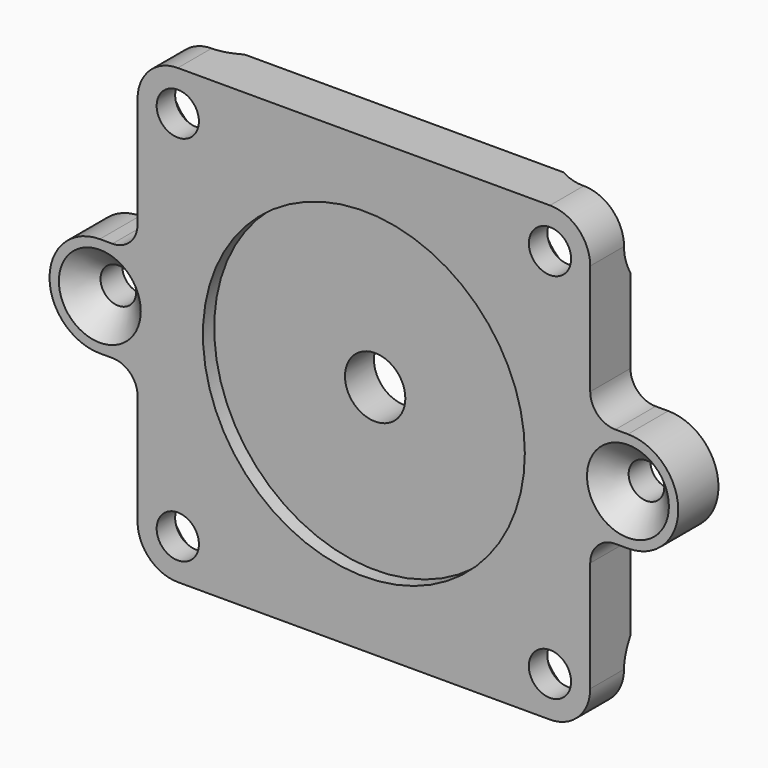
from build123d import *

# Parameters (mm, degrees)
F0_R     = 2.667
F0_R_2   = 2.2479
F0_R_3   = 3.81
F1_DEPTH = 6.35
F2_R     = 20.32
F2_R_2   = 3.81
F3_DEPTH = 1.778
F4_SIZE  = 2.921


# Not quite as in the source:
# - a fillet or chamfer that OpenCascade refuses, or shapes differently, is made with other operations: its cross-section is extruded or revolved along the edge and cut away or added


with BuildPart() as f1:
    # F0 (on Front) → F1 (new body)
    with BuildSketch(Plane.XZ):
        with BuildLine():
            Line((-23.495, -28.575), (23.495, -28.575))
            ThreePointArc((23.495, -28.575), (27.0871024484, -27.0871024484), (28.575, -23.495))
            Line((28.575, -23.495), (28.575, -9.525))
            ThreePointArc((28.575, -9.525), (29.5049359697, -7.2799359697), (31.75, -6.35))
            Line((31.75, -6.35), (33.3375, -6.35))
            ThreePointArc((33.3375, -6.35), (39.6875, 0), (33.3375, 6.35))
            Line((33.3375, 6.35), (31.75, 6.35))
            ThreePointArc((31.75, 6.35), (29.5049359697, 7.2799359697), (28.575, 9.525))
            Line((28.575, 9.525), (28.575, 23.495))
            ThreePointArc((28.575, 23.495), (27.0871024484, 27.0871024484), (23.495, 28.575))
            Line((23.495, 28.575), (-23.495, 28.575))
            ThreePointArc((-23.495, 28.575), (-27.0871024484, 27.0871024484), (-28.575, 23.495))
            Line((-28.575, 23.495), (-28.575, 9.525))
            ThreePointArc((-28.575, 9.525), (-29.5049359697, 7.2799359697), (-31.75, 6.35))
            Line((-31.75, 6.35), (-33.3375, 6.35))
            ThreePointArc((-33.3375, 6.35), (-39.6875, 0), (-33.3375, -6.35))
            Line((-33.3375, -6.35), (-31.75, -6.35))
            ThreePointArc((-31.75, -6.35), (-29.5049359697, -7.2799359697), (-28.575, -9.525))
            Line((-28.575, -9.525), (-28.575, -23.495))
            ThreePointArc((-28.575, -23.495), (-27.0871024484, -27.0871024484), (-23.495, -28.575))
        make_face()
        with Locations((-23.495, -23.495)):
            Circle(F0_R, mode=Mode.SUBTRACT)
        with Locations((23.495, -23.495)):
            Circle(F0_R, mode=Mode.SUBTRACT)
        with Locations((-33.3375, 0)):
            Circle(F0_R_2, mode=Mode.SUBTRACT)
        with Locations((-23.495, 23.495)):
            Circle(F0_R, mode=Mode.SUBTRACT)
        Circle(F0_R_3, mode=Mode.SUBTRACT)
        with Locations((33.3375, 0)):
            Circle(F0_R_2, mode=Mode.SUBTRACT)
        with Locations((23.495, 23.495)):
            Circle(F0_R, mode=Mode.SUBTRACT)
    extrude(amount=F1_DEPTH)

    # F2 (on face) → F3 (cut)
    with BuildSketch(Plane.XZ.offset(6.35)):
        Circle(F2_R)
        Circle(F2_R_2, mode=Mode.SUBTRACT)
        Circle(F2_R)
    extrude(amount=-F3_DEPTH, mode=Mode.SUBTRACT)

    # F4
    f4_edges = [f1.edges().sort_by_distance(p)[0] for p in [
        (-35.5854, -6.35, 0),
        (31.0896, -6.35, 0),
    ]]
    chamfer(f4_edges, length=F4_SIZE)

    # F5: chamfer of 3.429 on 4 edges, made by hand

    # F5_s1 → F5_t2 (revolve, cut)
    with BuildSketch(Plane.XY.offset(23.495)):
        Polygon((26.162, -3.429), (29.591, 0), (26.162, 0), align=None)
    revolve(axis=Axis((23.495, 0, 23.495), (0, -1, 0)), mode=Mode.SUBTRACT)

    # F5_s3 → F5_t4 (revolve, cut)
    with BuildSketch(Plane.XY.offset(23.495)):
        Polygon((-20.828, -3.429), (-17.399, 0), (-20.828, 0), align=None)
    revolve(axis=Axis((-23.495, 0, 23.495), (0, -1, 0)), mode=Mode.SUBTRACT)

    # F5_s5 → F5_t6 (revolve, cut)
    with BuildSketch(Plane.XY.offset(-23.495)):
        Polygon((26.162, -3.429), (29.591, 0), (26.162, 0), align=None)
    revolve(axis=Axis((23.495, 0, -23.495), (0, -1, 0)), mode=Mode.SUBTRACT)

    # F5_s7 → F5_t8 (revolve, cut)
    with BuildSketch(Plane.XY.offset(-23.495)):
        Polygon((-20.828, -3.429), (-17.399, 0), (-20.828, 0), align=None)
    revolve(axis=Axis((-23.495, 0, -23.495), (0, -1, 0)), mode=Mode.SUBTRACT)


solid = f1.part
